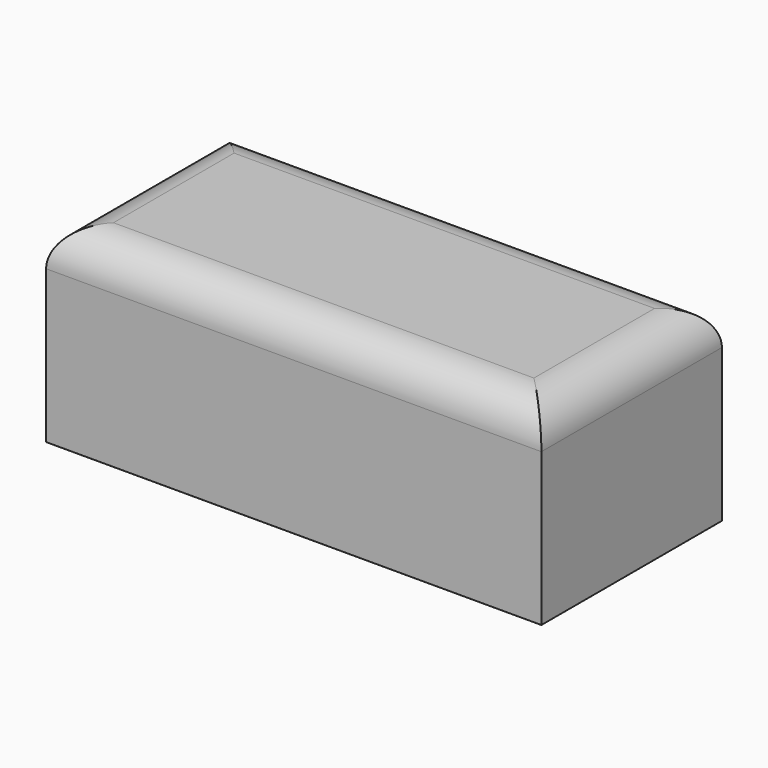
from build123d import *

# Parameters (mm, degrees)
F0_W     = 66.169410944
F0_H     = 30.1459496841
F1_DEPTH = 25.4
F6_R     = 3.4499508962
F7_DEPTH = 1.7
F8_R     = 5
F9_R     = 0.0241421356


# Not quite as in the source:
# - the program builds the solid bodies; features that only make, move or delete a surface that nothing else refers to are left out


with BuildPart() as f1:
    # F0 (on Top) → F1 (new body)
    with BuildSketch(Plane.XY):
        with Locations((1.8959715962, -3.7919436581)):
            Rectangle(F0_W, F0_H)
    extrude(amount=F1_DEPTH)

    # F6 (on face) → F7 (join)
    with BuildSketch(Plane(origin=(0, 0, 0), x_dir=(1, 0, 0), z_dir=(0, 0, -1))):
        with Locations((-15.3637295589, -6.2752226368)):
            Circle(F6_R)
    extrude(amount=F7_DEPTH)

    # F8
    f8_edges = [f1.edges().sort_by_distance(p)[0] for p in [
        (1.895972, 11.281031, 25.4),
        (-31.188734, -3.791944, 25.4),
        (1.895972, -18.864919, 25.4),
        (34.980677, -3.791944, 25.4),
    ]]
    fillet(f8_edges, radius=F8_R)

    # F9
    f9_edges = [f1.edges().sort_by_distance(p)[0] for p in [
        (1.895972, 11.281031, 0),
        (34.980677, -3.791944, 0),
        (-31.188734, -3.791944, 0),
        (1.895972, -18.864919, 0),
        (-18.81368, 6.275223, 0),
    ]]
    fillet(f9_edges, radius=F9_R)


solid = f1.part
